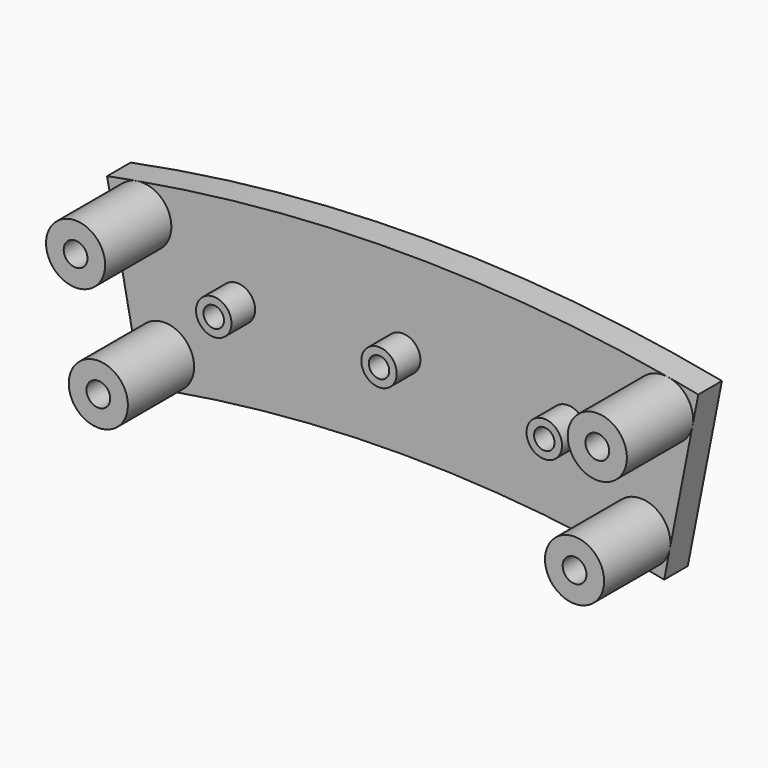
from build123d import *

# Parameters (mm, degrees)
F1_DEPTH = 6.35
F2_R     = 6.35
F3_DEPTH = 17.78
F5_D     = 5.1054
F6_R     = 3.81
F7_DEPTH = 6.35
F9_D     = 4.4


# Not quite as in the source:
# - a pattern or mirror of a feature is missing from the dataset's text; its kind, count and spacing are read off the source's solid


with BuildPart() as f1:
    # F0 (on Front) → F1 (new body)
    with BuildSketch(Plane.XZ):
        with BuildLine():
            Line((56.1730769231, 286.6478596274), (63.5, 324.0367108832))
            ThreePointArc((63.5, 324.0367108832), (0, 330.2), (-63.5, 324.0367108832))
            Line((-63.5, 324.0367108832), (-56.1730769231, 286.6478596274))
            ThreePointArc((-56.1730769231, 286.6478596274), (0, 292.1), (56.1730769231, 286.6478596274))
        make_face()
    extrude(amount=F1_DEPTH)

    # F2 (on face) → F3 (join)
    with BuildSketch(Plane.XZ.offset(6.35)):
        with Locations((-51.149763091, 294.0341888892)):
            Circle(F2_R)
        with Locations((-56.0353976971, 318.9652907527)):
            Circle(F2_R)
    f3 = extrude(amount=F3_DEPTH)

    # F3_copies: F3 across plane
    add(f3.mirror(Plane(origin=(0, 0, 0), x_dir=(0, 0, 1), z_dir=(1, 0, 0))))

    # F5 (through all)
    with Locations(Plane.XZ.offset(24.13)):
        with Locations((-56.0353976971, 318.9652907527), (-51.149763091, 294.0341888892)):
            f5 = Hole(F5_D / 2)

    # F5_copies: F5 across plane
    add(f5.mirror(Plane(origin=(0, 0, 0), x_dir=(0, 0, 1), z_dir=(1, 0, 0))), mode=Mode.SUBTRACT)

    # F6 (on face) → F7 (join)
    with BuildSketch(Plane.XZ.offset(6.35)):
        with Locations((0, 311.15)):
            Circle(F6_R)
        with Locations((-35.501895386, 309.118)):
            Circle(F6_R)
        with Locations((35.501895386, 309.118)):
            Circle(F6_R)
    extrude(amount=F7_DEPTH)

    # F9 (through all)
    with Locations(Plane.XZ.offset(12.7)):
        with Locations((-35.501895386, 309.118), (0, 311.15), (35.501895386, 309.118)):
            Hole(F9_D / 2)


solid = f1.part
